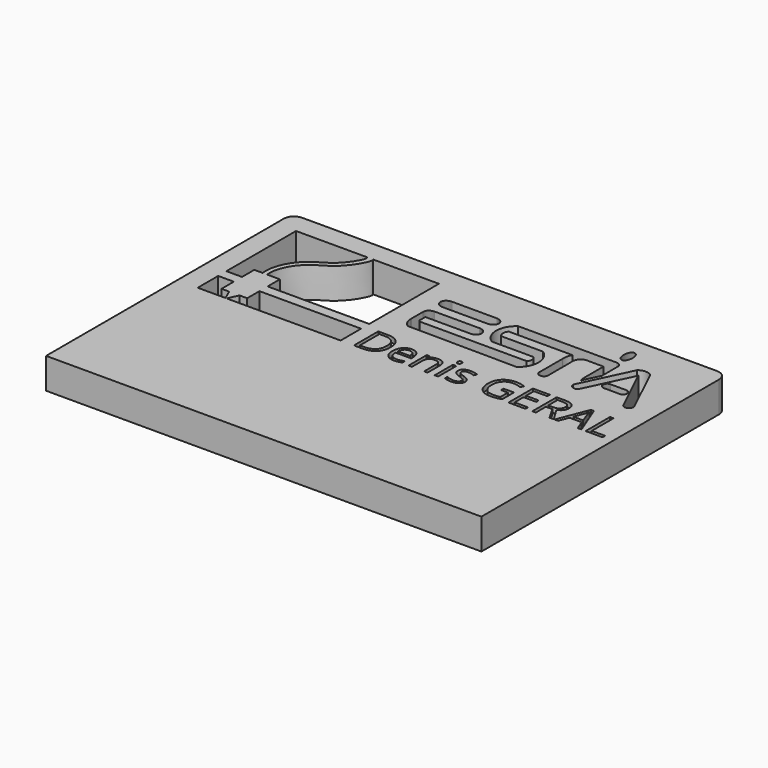
from build123d import *

# Parameters (mm, degrees)
F1_DEPTH     = 6
F2_TEXT_SIZE = 8.3333333333
F3_DEPTH     = 1


# Not quite as in the source:
# - Text() gives the source's letters only with a copy of the font that has no kerning and outlines rounded to 1/6400 em; it was checked with that copy


with BuildPart() as f1:
    # F0 (on Top) → F1 (new body)
    with BuildSketch(Plane.XY):
        with BuildLine():
            Line((-180.8656862974, -25.9791432917), (-261.8656862974, -25.9791432917))
            ThreePointArc((-261.8656862974, -25.9791432917), (-263.2798998598, -26.5649297293), (-263.8656862974, -27.9791432917))
            Line((-263.8656862974, -27.9791432917), (-263.8656862974, -85.9791432917))
            Line((-263.8656862974, -85.9791432917), (-178.8656862974, -85.9791432917))
            Line((-178.8656862974, -85.9791432917), (-178.8656862974, -27.9791432917))
            ThreePointArc((-178.8656862974, -27.9791432917), (-179.451472735, -26.5649297293), (-180.8656862974, -25.9791432917))
        make_face()
        Polygon((-259.8656862974, -53.9737103879), (-259.8656862974, -48.9737103879), (-256.8148994446, -48.9737103879), (-256.8148994446, -51.9737103879), (-255.3148994446, -51.9737103879), (-254.4423043728, -53.9737103879), align=None, mode=Mode.SUBTRACT)
        Polygon((-231.9663017988, -53.9737103879), (-254.2182207108, -53.9737103879), (-253.3148994446, -51.9737103879), (-251.8148994446, -51.9737103879), (-251.8148994446, -48.9737103879), (-231.9663017988, -48.9737103879), align=None, mode=Mode.SUBTRACT)
        with BuildLine():
            Line((-259.8656862974, -46.9737103879), (-259.8656862974, -29.9791432917))
            Line((-259.8656862974, -29.9791432917), (-245.9159940481, -29.9791432917))
            add(Edge.make_bspline(
                [(-255.1909685135, -43.9737103879), (-255.3791510604, -42.7416796501), (-254.8081738778, -39.5758147818), (-251.703943045, -36.1005307429), (-248.1297937931, -34.7922819685), (-245.5223963122, -30.5574073429), (-245.9159940481, -29.9791432917)],
                knots=[0, 0, 0, 0, 0.2459348193, 0.4965046927, 0.7440326327, 1, 1, 1, 1], degree=3))
            Line((-255.1909685135, -43.9737103879), (-256.8148994446, -43.9737103879))
            Line((-256.8148994446, -43.9737103879), (-256.8148994446, -46.9737103879))
            Line((-256.8148994446, -46.9737103879), (-259.8656862974, -46.9737103879))
        make_face(mode=Mode.SUBTRACT)
        with BuildLine():
            Line((-244.8035869415, -29.9791432917), (-231.9663017988, -29.9791432917))
            Line((-231.9663017988, -29.9791432917), (-231.9663017988, -46.9737103879))
            Line((-231.9663017988, -46.9737103879), (-251.8148994446, -46.9737103879))
            Line((-251.8148994446, -46.9737103879), (-251.8148994446, -43.9737103879))
            Line((-251.8148994446, -43.9737103879), (-254.3148994446, -43.9737103879))
            add(Edge.make_bspline(
                [(-254.3148994446, -43.9737103879), (-254.4993357491, -42.7662062911), (-253.7351079972, -39.7472627584), (-250.7864712115, -36.7626023965), (-247.0853364126, -35.282964803), (-244.3914240238, -30.5846828484), (-244.8035869415, -29.9791432917)],
                knots=[0, 0, 0, 0, 0.2410388741, 0.4793497451, 0.7319591875, 1, 1, 1, 1], degree=3))
        make_face(mode=Mode.SUBTRACT)
        Polygon((-226.841587332, -35.6446195563), (-226.9569276525, -35.6316028818), (-227.0705037525, -35.6100198033), (-227.181451143, -35.5800362463), (-227.288927052, -35.5418815728), (-227.392115568, -35.4958379133), (-227.4902324025, -35.4422597883), (-227.5825239375, -35.3815571538), (-227.6682927525, -35.3141919723), (-227.746887528, -35.2406732598), (-227.817705903, -35.1615675633), (-227.880210858, -35.0774680998), (-227.933927667, -34.9890200928), (-227.9784496125, -34.8968977218), (-228.013429413, -34.8017987883), (-228.0386095125, -34.7044471923), (-228.053792553, -34.6055870268), (-228.058865568, -34.5059680998), (-228.053792553, -34.4063491728), (-228.0386095125, -34.3074890073), (-228.013429413, -34.2101374113), (-227.9784496125, -34.1150384778), (-227.933927667, -34.0229161068), (-227.880210858, -33.9344680998), (-227.817705903, -33.8503714938), (-227.746887528, -33.7712657973), (-227.6682927525, -33.6977442273), (-227.5825239375, -33.6303820938), (-227.4902324025, -33.5696764113), (-227.392115568, -33.5161011438), (-227.288927052, -33.4700574843), (-227.181451143, -33.4318999533), (-227.0705037525, -33.4019163963), (-226.9569276525, -33.3803333178), (-226.841589618, -33.3673166433), (-226.725365568, -33.3629680998), (-217.962365568, -33.3629680998), (-217.846143042, -33.3673166433), (-217.730807103, -33.3803333178), (-217.617232527, -33.4019163963), (-217.506281517, -33.4318999533), (-217.3988054175, -33.4700574843), (-217.295615568, -33.5161011438), (-217.197503877, -33.5696764113), (-217.105208532, -33.6303820938), (-217.019443527, -33.6977442273), (-216.940845132, -33.7712657973), (-216.870026757, -33.8503714938), (-216.807521802, -33.9344680998), (-216.7538086125, -34.0229161068), (-216.709285143, -34.1150384778), (-216.674303247, -34.2101374113), (-216.6491288625, -34.3074890073), (-216.6339422025, -34.4063491728), (-216.628865568, -34.5059680998), (-216.6339422025, -34.6055870268), (-216.6491288625, -34.7044471923), (-216.674303247, -34.8017987883), (-216.709285143, -34.8968977218), (-216.7538086125, -34.9890200928), (-216.807521802, -35.0774680998), (-216.870026757, -35.1615675633), (-216.940845132, -35.2406732598), (-217.019443527, -35.3141919723), (-217.105208532, -35.3815571538), (-217.197503877, -35.4422597883), (-217.295615568, -35.4958379133), (-217.3988054175, -35.5418815728), (-217.506281517, -35.5800362463), (-217.617232527, -35.6100198033), (-217.730807103, -35.6316028818), (-217.846143042, -35.6446195563), (-217.962365568, -35.6489680998), (-226.725365568, -35.6489680998), align=None, mode=Mode.SUBTRACT)
        with BuildLine():
            Line((-226.725365568, -39.8399680998), (-226.725365568, -41.1734680998))
            ThreePointArc((-226.725365568, -41.1734680998), (-226.6137732517, -41.4428757835), (-226.344365568, -41.5544680998))
            Line((-226.344365568, -41.5544680998), (-205.5798665256, -41.5544680998))
            ThreePointArc((-205.5798665256, -41.5544680998), (-205.1949039404, -40.6972180998), (-205.5798665256, -39.8399680998))
            Line((-205.5798665256, -39.8399680998), (-213.771365568, -39.8399680998))
            ThreePointArc((-213.771365568, -39.8399680998), (-215.485867876, -36.6014680998), (-213.771365568, -33.3629680998))
            Line((-213.771365568, -33.3629680998), (-194.530865568, -33.3629680998))
            ThreePointArc((-194.530865568, -33.3629680998), (-193.857346359, -33.6419488908), (-193.578365568, -34.3154680998))
            Line((-193.578365568, -34.3154680998), (-193.578365568, -38.1254680998))
            Line((-193.578365568, -38.1254680998), (-195.107321616, -41.3532579993))
            ThreePointArc((-195.107321616, -41.3532579993), (-195.2573582512, -40.8936448771), (-195.292865568, -40.4114680998))
            Line((-195.292865568, -40.4114680998), (-195.292865568, -35.6489680998))
            Line((-195.292865568, -35.6489680998), (-198.721865568, -35.6489680998))
            ThreePointArc((-198.721865568, -35.6489680998), (-199.7831558124, -36.3252899287), (-200.055365568, -37.5539680998))
            Line((-200.055365568, -37.5539680998), (-200.055365568, -43.0784680998))
            ThreePointArc((-200.055365568, -43.0784680998), (-200.912615568, -44.0361427928), (-201.769865568, -43.0784680998))
            Line((-201.769865568, -43.0784680998), (-201.769865568, -37.5539680998))
            ThreePointArc((-201.769865568, -37.5539680998), (-201.7127679043, -36.5747876326), (-201.388865568, -35.6489680998))
            Line((-201.388865568, -35.6489680998), (-213.771365568, -35.6489680998))
            ThreePointArc((-213.771365568, -35.6489680998), (-214.152365568, -36.6014680998), (-213.771365568, -37.5539680998))
            Line((-213.771365568, -37.5539680998), (-205.5798673925, -37.5539680998))
            ThreePointArc((-205.5798673925, -37.5539680998), (-203.8653650846, -40.7924680998), (-205.5798673925, -44.0309680998))
            Line((-205.5798673925, -44.0309680998), (-227.0117253065, -43.8363179564))
            ThreePointArc((-227.0117253065, -43.8363179564), (-227.7566419514, -42.9417156207), (-228.0591644931, -41.8175740555))
            ThreePointArc((-228.0591644931, -41.8175740555), (-228.0621973716, -41.6860438019), (-228.058865568, -41.5545207808))
            Line((-228.058865568, -41.5545207808), (-228.058865568, -38.6969680998))
            Line((-228.058865568, -38.6969680998), (-228.053792553, -38.5973535543))
            Line((-228.053792553, -38.5973535543), (-228.0386095125, -38.4984918648))
            Line((-228.0386095125, -38.4984918648), (-228.013429413, -38.4011402688))
            Line((-228.013429413, -38.4011402688), (-227.9784496125, -38.3060428593))
            Line((-227.9784496125, -38.3060428593), (-227.933927667, -38.2139191548))
            Line((-227.933927667, -38.2139191548), (-227.880210858, -38.1254680998))
            Line((-227.880210858, -38.1254680998), (-227.817705903, -38.0413714938))
            Line((-227.817705903, -38.0413714938), (-227.746887528, -37.9622644638))
            Line((-227.746887528, -37.9622644638), (-227.6682927525, -37.8887470848))
            Line((-227.6682927525, -37.8887470848), (-227.5825239375, -37.8213805698))
            Line((-227.5825239375, -37.8213805698), (-227.4902324025, -37.7606792688))
            Line((-227.4902324025, -37.7606792688), (-227.392115568, -37.7071011438))
            Line((-227.392115568, -37.7071011438), (-227.288927052, -37.6610574843))
            Line((-227.288927052, -37.6610574843), (-227.181451143, -37.6228999533))
            Line((-227.181451143, -37.6228999533), (-227.0705037525, -37.5929192538))
            Line((-227.0705037525, -37.5929192538), (-226.9569276525, -37.5713376993))
            Line((-226.9569276525, -37.5713376993), (-226.841589618, -37.5583166433))
            Line((-226.841589618, -37.5583166433), (-226.725365568, -37.5539680998))
            Line((-226.725365568, -37.5539680998), (-217.962365568, -37.5539680998))
            Line((-217.962365568, -37.5539680998), (-217.846143042, -37.5583166433))
            Line((-217.846143042, -37.5583166433), (-217.730807103, -37.5713376993))
            Line((-217.730807103, -37.5713376993), (-217.617232527, -37.5929192538))
            Line((-217.617232527, -37.5929192538), (-217.506281517, -37.6228999533))
            Line((-217.506281517, -37.6228999533), (-217.3988054175, -37.6610574843))
            Line((-217.3988054175, -37.6610574843), (-217.295615568, -37.7071011438))
            Line((-217.295615568, -37.7071011438), (-217.197503877, -37.7606792688))
            Line((-217.197503877, -37.7606792688), (-217.105208532, -37.8213805698))
            Line((-217.105208532, -37.8213805698), (-217.019443527, -37.8887470848))
            Line((-217.019443527, -37.8887470848), (-216.940845132, -37.9622644638))
            Line((-216.940845132, -37.9622644638), (-216.870026757, -38.0413714938))
            Line((-216.870026757, -38.0413714938), (-216.807521802, -38.1254680998))
            Line((-216.807521802, -38.1254680998), (-216.7538086125, -38.2139191548))
            Line((-216.7538086125, -38.2139191548), (-216.709285143, -38.3060428593))
            Line((-216.709285143, -38.3060428593), (-216.674303247, -38.4011402688))
            Line((-216.674303247, -38.4011402688), (-216.6491288625, -38.4984918648))
            Line((-216.6491288625, -38.4984918648), (-216.6339422025, -38.5973535543))
            Line((-216.6339422025, -38.5973535543), (-216.628865568, -38.6969680998))
            Line((-216.628865568, -38.6969680998), (-216.6339422025, -38.7965898843))
            Line((-216.6339422025, -38.7965898843), (-216.6491288625, -38.8954515738))
            Line((-216.6491288625, -38.8954515738), (-216.674303247, -38.9927987883))
            Line((-216.674303247, -38.9927987883), (-216.709285143, -39.0879005793))
            Line((-216.709285143, -39.0879005793), (-216.7538086125, -39.1800242838))
            Line((-216.7538086125, -39.1800242838), (-216.807521802, -39.2684680998))
            Line((-216.807521802, -39.2684680998), (-216.870026757, -39.3525675633))
            Line((-216.870026757, -39.3525675633), (-216.940845132, -39.4316732598))
            Line((-216.940845132, -39.4316732598), (-217.019443527, -39.5051963538))
            Line((-217.019443527, -39.5051963538), (-217.105208532, -39.5725571538))
            Line((-217.105208532, -39.5725571538), (-217.197503877, -39.6332597883))
            Line((-217.197503877, -39.6332597883), (-217.295615568, -39.6868363893))
            Line((-217.295615568, -39.6868363893), (-217.3988054175, -39.7328802393))
            Line((-217.3988054175, -39.7328802393), (-217.506281517, -39.7710391038))
            Line((-217.506281517, -39.7710391038), (-217.617232527, -39.8010198033))
            Line((-217.617232527, -39.8010198033), (-217.730807103, -39.8226057393))
            Line((-217.730807103, -39.8226057393), (-217.846143042, -39.8356224138))
            Line((-217.846143042, -39.8356224138), (-217.962365568, -39.8399680998))
            Line((-217.962365568, -39.8399680998), (-226.725365568, -39.8399680998))
        make_face(mode=Mode.SUBTRACT)
        Polygon((-190.894070073, -41.1703869528), (-190.9633943565, -41.1611678958), (-191.031660603, -41.1458810328), (-191.098351224, -41.1246410448), (-191.1629518695, -41.0976123333), (-191.224974288, -41.0649994953), (-191.2839475635, -41.0270497998), (-191.3394238305, -40.9840524258), (-191.390978655, -40.9363342713), (-191.4382171305, -40.8842605248), (-191.4807843555, -40.8282245688), (-191.5183547655, -40.7686555998), (-191.5506433725, -40.7060052933), (-191.577400431, -40.6407506613), (-191.598428202, -40.5733898613), (-191.6135639985, -40.5044334333), (-191.622688377, -40.4344071573), (-191.625740568, -40.3638430998), (-191.622688377, -40.2932790423), (-191.6135639985, -40.2232527663), (-191.598428202, -40.1542963383), (-191.577400431, -40.0869355383), (-191.5506433725, -40.0216809063), (-191.5183547655, -39.9590305998), (-191.4807843555, -39.8994616308), (-191.4382171305, -39.8434256748), (-191.390978655, -39.7913519283), (-191.3394238305, -39.7436337738), (-191.283950421, -39.7006363998), (-191.224974288, -39.6626867043), (-191.1629518695, -39.6300738663), (-191.098351224, -39.6030451548), (-191.031660603, -39.5818051668), (-190.9633943565, -39.5665183038), (-190.894070073, -39.5572992468), (-190.824211056, -39.5542180998), (-187.71239508, -39.5542180998), (-187.642536063, -39.5572992468), (-187.5732117795, -39.5665183038), (-187.5049426755, -39.5818051668), (-187.438254912, -39.6030451548), (-187.3736542665, -39.6300738663), (-187.311631848, -39.6626867043), (-187.252655715, -39.7006363998), (-187.1971823055, -39.7436337738), (-187.145627481, -39.7913519283), (-187.0983890055, -39.8434256748), (-187.0558217805, -39.8994616308), (-187.0182513705, -39.9590305998), (-186.9859627635, -40.0216809063), (-186.959205705, -40.0869355383), (-186.938177934, -40.1542963383), (-186.9230421375, -40.2232527663), (-186.913917759, -40.2932790423), (-186.910865568, -40.3638430998), (-186.913917759, -40.4344071573), (-186.9230421375, -40.5044334333), (-186.938177934, -40.5733898613), (-186.959205705, -40.6407519948), (-186.9859627635, -40.7060052933), (-187.0182513705, -40.7686555998), (-187.0558217805, -40.8282245688), (-187.0983890055, -40.8842605248), (-187.145627481, -40.9363342713), (-187.1971823055, -40.9840524258), (-187.2526585725, -41.0270497998), (-187.311631848, -41.0649994953), (-187.3736542665, -41.0976123333), (-187.438254912, -41.1246410448), (-187.504945533, -41.1458810328), (-187.5732117795, -41.1611678958), (-187.642536063, -41.1703869528), (-187.71239508, -41.1734680998), (-190.824211056, -41.1734680998), align=None, mode=Mode.SUBTRACT)
        with BuildLine():
            Line((-184.910615568, -43.8465606708), (-189.271465749, -34.6835415318))
            Line((-189.271465749, -34.6835415318), (-193.625990568, -43.8775995978))
            ThreePointArc((-193.625990568, -43.8775995978), (-194.6229966055, -43.9973439176), (-195.197615568, -43.1738314473))
            Line((-195.197615568, -43.1738314473), (-190.5532506654, -33.3758113587))
            ThreePointArc((-190.5532506654, -33.3758113587), (-189.2634011694, -32.9126942774), (-187.9721873595, -33.3719937993))
            Line((-187.9721873595, -33.3719937993), (-183.338990568, -43.1538020868))
            ThreePointArc((-183.338990568, -43.1538020868), (-183.8812568122, -44.0527019727), (-184.910615568, -43.8465606708))
        make_face(mode=Mode.SUBTRACT)
        Polygon((-193.5938442645, -30.4064915388), (-193.5828623205, -30.5380125483), (-193.578365568, -30.6707312313), (-193.580397441, -30.8036476533), (-193.588931841, -30.9357382578), (-193.6039133325, -31.0660065393), (-193.6252260915, -31.1934580878), (-193.652698287, -31.3171190673), (-193.686135228, -31.4360565993), (-193.7252751675, -31.5493578078), (-193.7698190205, -31.6561652523), (-193.8194294115, -31.7556620688), (-193.873731246, -31.8470955918), (-193.932311901, -31.9297678293), (-193.9947179865, -32.0030482263), (-194.0604785865, -32.0663845233), (-194.129096496, -32.1192823728), (-194.2000426965, -32.1613525833), (-194.2727824545, -32.1922692093), (-194.3467635105, -32.2117971738), (-194.421418746, -32.2197850293), (-194.4961844715, -32.2161777213), (-194.5704851865, -32.2010011578), (-194.643762726, -32.1743690673), (-194.715450162, -32.1364849038), (-194.785012761, -32.0876361318), (-194.8519127415, -32.0281949883), (-194.915644326, -31.9586148633), (-194.975728026, -31.8794221083), (-195.0316925445, -31.7912238468), (-195.0831225915, -31.6946919723), (-195.1296255465, -31.5905530518), (-195.1708497465, -31.4796121383), (-195.206472675, -31.3627005738), (-195.236229537, -31.2407138988), (-195.259893828, -31.1145849918), (-195.277282287, -30.9852701628), (-195.288269946, -30.8537491533), (-195.292763841, -30.7210276128), (-195.2907348255, -30.5881113813), (-195.2821947105, -30.4560175383), (-195.267215886, -30.3257551623), (-195.2459033175, -30.1983007563), (-195.2184282645, -30.0746369193), (-195.184994181, -29.9557022448), (-195.1458542415, -29.8423981788), (-195.101307531, -29.7355907343), (-195.05169714, -29.6360939178), (-194.9973953055, -29.5446634428), (-194.9388203655, -29.4619881573), (-194.8764114225, -29.3887106178), (-194.8106508225, -29.3253745113), (-194.742032913, -29.2724736138), (-194.6710867125, -29.2304034033), (-194.598344097, -29.1994867773), (-194.524363041, -29.1799588128), (-194.4497078055, -29.1719709573), (-194.3749449375, -29.1755813133), (-194.3006411745, -29.1907548288), (-194.227366683, -29.2173869193), (-194.155679247, -29.2552710828), (-194.0861164575, -29.3041229028), (-194.0192136195, -29.3635609983), (-193.955482035, -29.4331411233), (-193.895404431, -29.5123338783), (-193.839434007, -29.6005321398), (-193.78800396, -29.6970640143), (-193.741501005, -29.8012000773), (-193.7002796625, -29.9121497538), (-193.6646538765, -30.0290554128), (-193.6348970145, -30.1510420878), (-193.611235581, -30.2771709948), align=None, mode=Mode.SUBTRACT)
    extrude(amount=F1_DEPTH)

    # F2 (on face) → F3 (cut)
    with BuildSketch(Plane.XY.offset(6)):
        with Locations((-230.1804870367, -53.9737103879)):
            Text('Denis GERAL', F2_TEXT_SIZE, font='Open Sans', text_align=(TextAlign.LEFT, TextAlign.BOTTOM))
    extrude(amount=-F3_DEPTH, mode=Mode.SUBTRACT)


solid = f1.part
